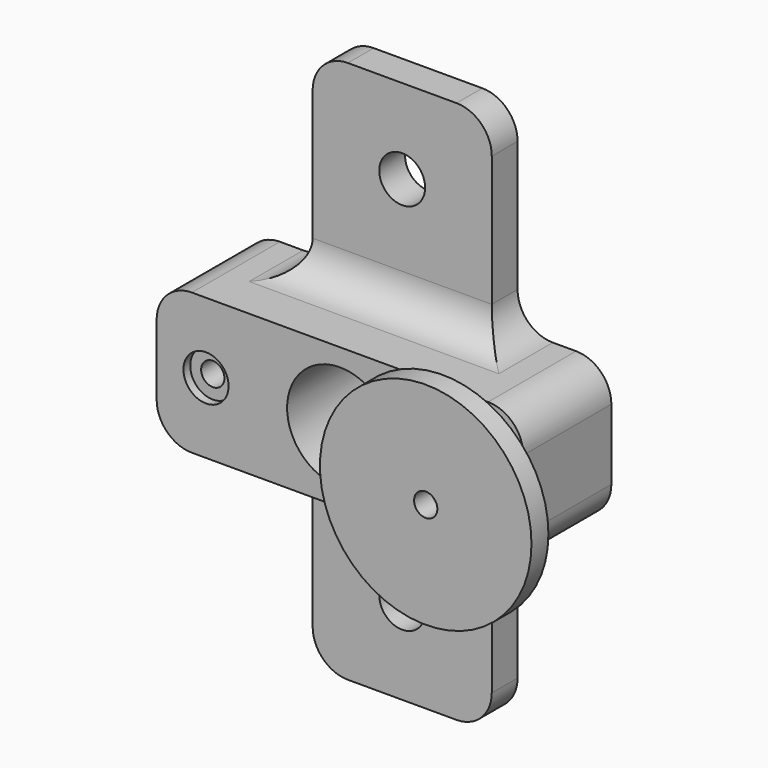
from build123d import *

# Parameters (mm, degrees)
F0_W     = 25.4
F0_H     = 28.5
F0_R     = 3.2512
F0_H_2   = 20
F0_R_2   = 7.5
F1_DEPTH = 4.572
F0_W_2   = 13.3
F0_R_3   = 1.65
F2_DEPTH = 15.6
F3_R     = 3.2
F3_R_2   = 1.65
F4_DEPTH = 1.2
F5_R     = 5
F7_R     = 15
F7_R_2   = 2.25
F7_R_3   = 1.65
F8_DEPTH = 3
F9_DEPTH = 0.6


# Not quite as in the source:
# - a length typed as a fraction of an inch, garbled in the dataset ("3 / 203.2 mm" for 3/8 in), is restored


with BuildPart() as f1:
    # F0 (on Front) → F1 (new body)
    with BuildSketch(Plane.XZ):
        with Locations((0, 24.25)):
            Rectangle(F0_W, F0_H)
        with Locations((0, 26.5)):
            Circle(F0_R, mode=Mode.SUBTRACT)
        with Locations((0, -24.25)):
            Rectangle(F0_W, F0_H)
        with Locations((0, -26.5)):
            Circle(F0_R, mode=Mode.SUBTRACT)
        Rectangle(F0_W, F0_H_2)
        Circle(F0_R_2, mode=Mode.SUBTRACT)
    extrude(amount=F1_DEPTH)

    # F0 (on Front) → F2 (join)
    with BuildSketch(Plane.XZ):
        with Locations((19.35, 0)):
            Rectangle(F0_W_2, F0_H_2)
        with Locations((19, 0)):
            Circle(F0_R_3, mode=Mode.SUBTRACT)
        with Locations((-19.35, 0)):
            Rectangle(F0_W_2, F0_H_2)
        with Locations((-19, 0)):
            Circle(F0_R_3, mode=Mode.SUBTRACT)
        Rectangle(F0_W, F0_H_2)
        Circle(F0_R_2, mode=Mode.SUBTRACT)
    extrude(amount=F2_DEPTH)

    # F3 (on face) → F4 (cut)
    with BuildSketch(Plane.XZ.offset(15.6)):
        with Locations((-19, 0)):
            Circle(F3_R)
        with Locations((-19, 0)):
            Circle(F3_R_2, mode=Mode.SUBTRACT)
        with Locations((19, 0)):
            Circle(F3_R)
        with Locations((19, 0)):
            Circle(F3_R_2, mode=Mode.SUBTRACT)
    extrude(amount=-F4_DEPTH, mode=Mode.SUBTRACT)

    # F5
    f5_edges = [f1.edges().sort_by_distance(p)[0] for p in [
        (0, -4.572, 10),
        (0, -4.572, -10),
        (26, -7.8, -10),
        (-26, -7.8, -10),
        (-26, -7.8, 10),
        (26, -7.8, 10),
        (-12.7, -2.286, 10),
        (12.7, -2.286, 10),
        (12.7, -2.286, -10),
        (-12.7, -2.286, -10),
        (12.7, -2.286, 38.5),
        (-12.7, -2.286, 38.5),
        (12.7, -2.286, -38.5),
        (-12.7, -2.286, -38.5),
    ]]
    fillet(f5_edges, radius=F5_R)


with BuildPart() as f8:
    # F7 (on offset) → F8 (new body)
    with BuildSketch(Plane.XZ.offset(21.15625)):
        with Locations((19, 0)):
            Circle(F7_R)
        with Locations((19, 0)):
            Circle(F7_R_2, mode=Mode.SUBTRACT)
        with Locations((19, 0)):
            Circle(F7_R_2)
        with Locations((19, 0)):
            Circle(F7_R_3, mode=Mode.SUBTRACT)
    extrude(amount=F8_DEPTH)

    # F7 (on offset) → F9 (join)
    with BuildSketch(Plane.XZ.offset(21.15625)):
        with Locations((19, 0)):
            Circle(F7_R_2)
        with Locations((19, 0)):
            Circle(F7_R_3, mode=Mode.SUBTRACT)
    extrude(amount=-F9_DEPTH)


solid = Compound([f1.part, f8.part])
